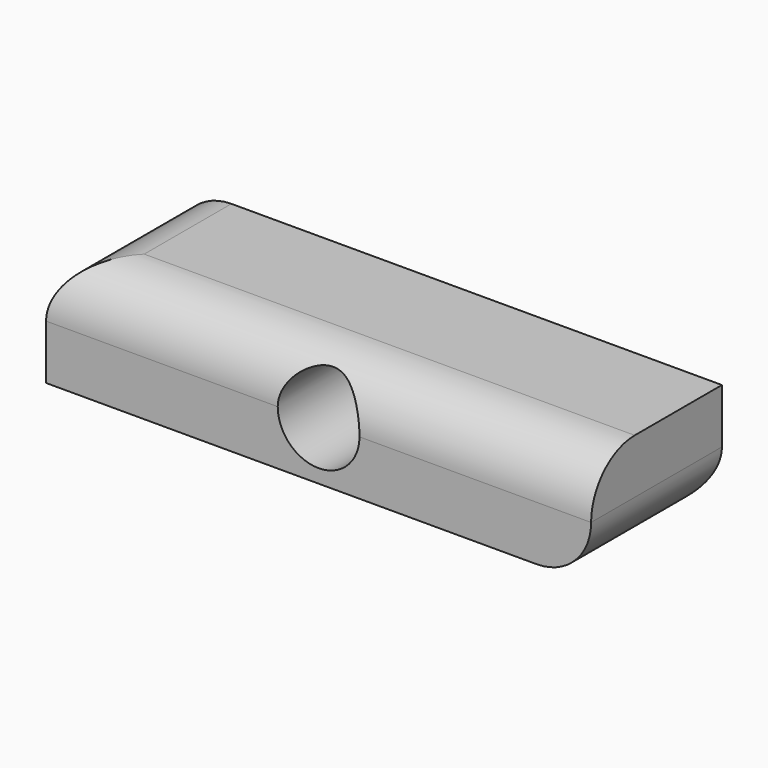
from build123d import *

# Parameters (mm, degrees)
F0_W        = 200
F0_H        = 40
F0_R        = 15
F1_DEPTH    = 30
F2_T1_DEPTH = 160
F2_T3_DEPTH = 300


# Not quite as in the source:
# - a fillet or chamfer that OpenCascade refuses, or shapes differently, is made with other operations: its cross-section is extruded or revolved along the edge and cut away or added


with BuildPart() as f1:
    # F0 (on Front) → F1 (new body, symmetric)
    with BuildSketch(Plane.XZ):
        with Locations((-100, -20)):
            Rectangle(F0_W, F0_H)
        with Locations((-100, -20)):
            Circle(F0_R, mode=Mode.SUBTRACT)
    extrude(amount=F1_DEPTH, both=True)

    # F2: fillet of radius 20 on 4 edges, made by hand

    # F2_s2 → F2_t1 (cut)
    with BuildSketch(Plane.XZ.offset(-80)):
        with BuildLine():
            ThreePointArc((-180, 0), (-194.1421356237, -5.8578643763), (-200, -20))
            Line((-200, -20), (-200, 0))
            Line((-200, 0), (-180, 0))
        make_face()
        with BuildLine():
            ThreePointArc((0, -20), (-5.8578643763, -34.1421356237), (-20, -40))
            Line((-20, -40), (0, -40))
            Line((0, -40), (0, -20))
        make_face()
    extrude(amount=F2_T1_DEPTH, mode=Mode.SUBTRACT)

    # F2_s4 → F2_t3 (cut)
    with BuildSketch(Plane.YZ.offset(-250)):
        with BuildLine():
            ThreePointArc((-10, 0), (-24.1421356237, -5.8578643763), (-30, -20))
            Line((-30, -20), (-30, 0))
            Line((-30, 0), (-10, 0))
        make_face()
        with BuildLine():
            ThreePointArc((10, -40), (24.1421356237, -34.1421356237), (30, -20))
            Line((30, -20), (30, -40))
            Line((30, -40), (10, -40))
        make_face()
    extrude(amount=F2_T3_DEPTH, mode=Mode.SUBTRACT)


solid = f1.part
